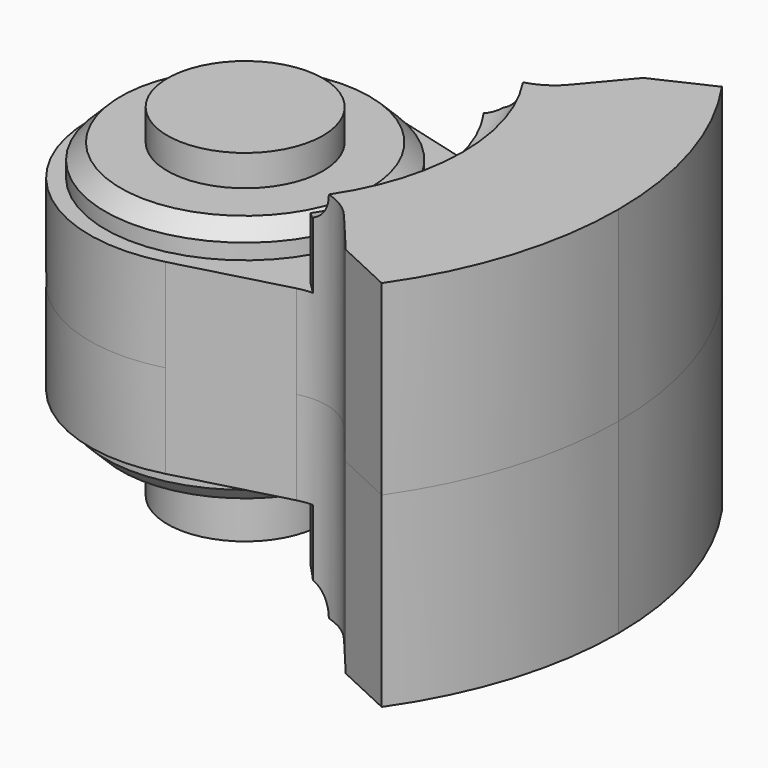
from build123d import *
from build123d import SkipClean  # not in build123d's __all__

# Parameters (mm, degrees)
F1_DEPTH       = 4.7625
F3_DEPTH       = 2.38125
F4_R           = 0.79375
F8_DEPTH       = 25.4
F10_R          = 3.571875
F11_DEPTH      = 3.175
F13_SIZE2      = 0.396875
F13_SIZE       = 0.396875
F12_R          = 1.984375
F15_DEPTH      = 3.96875
F15_DEPTH_BACK = 4.7625
F16_R          = 1.5875
F17_DEPTH      = 25.4


with BuildPart() as f1:
    # F0 (on Top) → F1 (new body)
    with BuildSketch(Plane.XY):
        with BuildLine():
            Line((7.8270786991, 5.4279336804), (6.3629416959, 4.7451953832))
            Line((6.3629416959, 4.7451953832), (5.4090072937, 3.6083406323))
            ThreePointArc((5.4090072937, 3.6083406323), (4.670282197, 3.1147403034), (3.7820365062, 3.0953587134))
            Line((3.7820365062, 3.0953587134), (1.0271880853, 3.8335181231))
            ThreePointArc((1.0271880853, 3.8335181231), (-2.4160219214, 3.1486210693), (-3.96875, 0))
            Line((-3.96875, 0), (9.525, 0))
            ThreePointArc((9.525, 0), (9.0906146549, 2.8436508568), (7.8270786991, 5.4279336804))
        make_face()
    extrude(amount=F1_DEPTH)

    # F2 (on face) → F3 (cut)
    with BuildSketch(Plane.XY.offset(4.7625)):
        with BuildLine():
            Line((3.5700563335, 3.1521586295), (1.0271880853, 3.8335181231))
            ThreePointArc((1.0271880853, 3.8335181231), (-2.4160219214, 3.1486210693), (-3.96875, 0))
            Line((-3.96875, 0), (4.7625, 0))
            ThreePointArc((4.7625, 0), (4.4544247405, 1.6850835234), (3.5700563335, 3.1521586295))
        make_face()
    extrude(amount=-F3_DEPTH, mode=Mode.SUBTRACT)

    # F6: sweep along a path in F5
    with BuildLine(Plane.XY.offset(4.7625)) as f6_path:
        ThreePointArc((4.7625, 0), (4.4544247405, 1.6850835234), (3.5700563335, 3.1521586295))
    # F4 (on Front) → F6 (sweep, cut)
    with BuildSketch(Plane.XZ):
        with Locations((4.7625, 4.7625)):
            Circle(F4_R)
    sweep(path=f6_path.line, mode=Mode.SUBTRACT)

    # F7 (on face) → F8 (cut)
    with BuildSketch(Plane.XY.offset(2.38125)):
        with BuildLine():
            ThreePointArc((3.5700563335, 3.1521586295), (3.7304279124, 2.9606272714), (3.880535973, 2.7609503459))
            Line((3.880535973, 2.7609503459), (4.1611689768, 3.0415833497))
            Line((4.1611689768, 3.0415833497), (4.1606985033, 3.6664465442))
            Line((4.1606985033, 3.6664465442), (2.6852940209, 3.5708183423))
            Line((2.6852940209, 3.5708183423), (3.1285953124, 3.2704477536))
            Line((3.1285953124, 3.2704477536), (3.5700563335, 3.1521586295))
        make_face()
    extrude(amount=F8_DEPTH, mode=Mode.SUBTRACT)

    # F9: F1 across face


with BuildPart() as f1_1:
    add(f1.part, clean=False)
    with SkipClean():  # cleaning this boolean's faces spoils the solid; the shape is the same uncleaned
        add(f1.part.mirror(Plane(origin=(3.9033700373, 0, 1.7817262918), x_dir=(1, 0, 0), z_dir=(0, -1, 0))), clean=False)

    # F10 (on Top) → F11 (join)
    with BuildSketch(Plane.XY):
        Circle(F10_R)
    extrude(amount=F11_DEPTH)

    # F13
    f13_edges = [f1_1.edges().sort_by_distance(p)[0] for p in [
        (-3.571875, 0, 3.175),
    ]]
    chamfer(f13_edges, length=F13_SIZE, length2=F13_SIZE2)

    # F14: F1 across plane


with BuildPart() as f1_2:
    add(f1_1.part, clean=False)
    add(f1_1.part.mirror(Plane.XY), clean=False)

    # F12 (on Top) → F15 (join, two sides)
    with BuildSketch(Plane.XY) as f15_sk:
        Circle(F12_R)
    with SkipClean():  # cleaning this boolean's faces spoils the solid; the shape is the same uncleaned
        extrude(amount=F15_DEPTH)
        extrude(f15_sk.sketch, amount=-F15_DEPTH_BACK)

    # F16 (on Right) → F17 (cut)
    with BuildSketch(Plane.YZ):
        Circle(F16_R)
    with SkipClean():  # cleaning this boolean's faces spoils the solid; the shape is the same uncleaned
        extrude(amount=-F17_DEPTH, mode=Mode.SUBTRACT)


solid = f1_2.part
